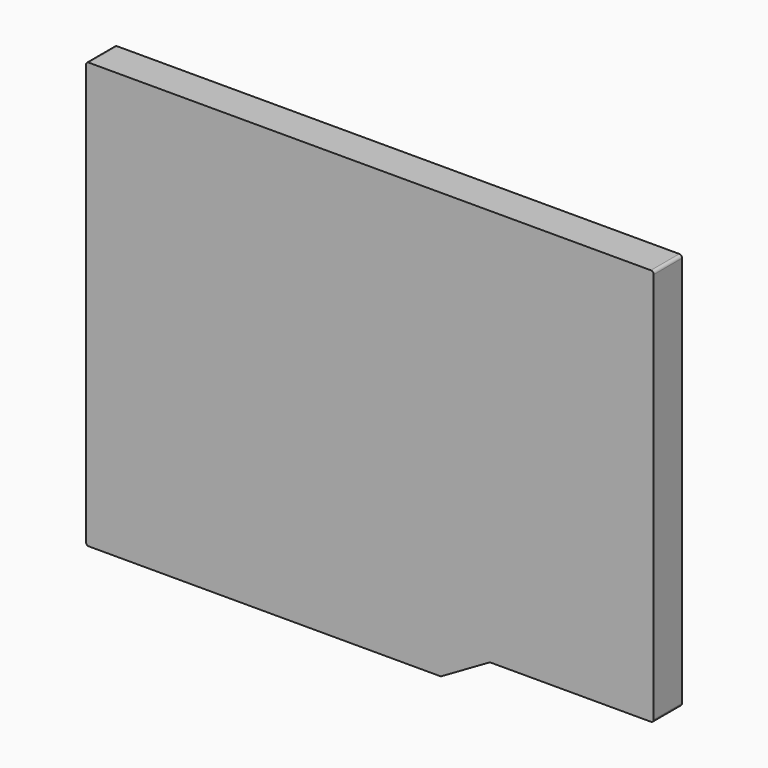
from build123d import *

# Parameters (mm, degrees)
F0_W     = 400
F0_H     = 300
F1_DEPTH = 25
F3_DEPTH = 25.001
F4_R     = 2


with BuildPart() as f1:
    # F0 (on Front) → F1 (new body)
    with BuildSketch(Plane.XZ):
        Rectangle(F0_W, F0_H)
    extrude(amount=F1_DEPTH)

    # F2 (on face) → F3 (cut, through all)
    with BuildSketch(Plane.XZ.offset(25)):
        Polygon((84.6410161514, -130), (50, -150), (200, -150), (200, -130), align=None)
    extrude(amount=-F3_DEPTH, mode=Mode.SUBTRACT)

    # F4
    f4_edges = [f1.edges().sort_by_distance(p)[0] for p in [
        (200, -12.5, 150),
        (200, -12.5, -130),
        (-200, -12.5, -150),
        (-200, -12.5, 150),
        (50, -12.5, -150),
        (84.641016, -12.5, -130),
    ]]
    fillet(f4_edges, radius=F4_R)


solid = f1.part
